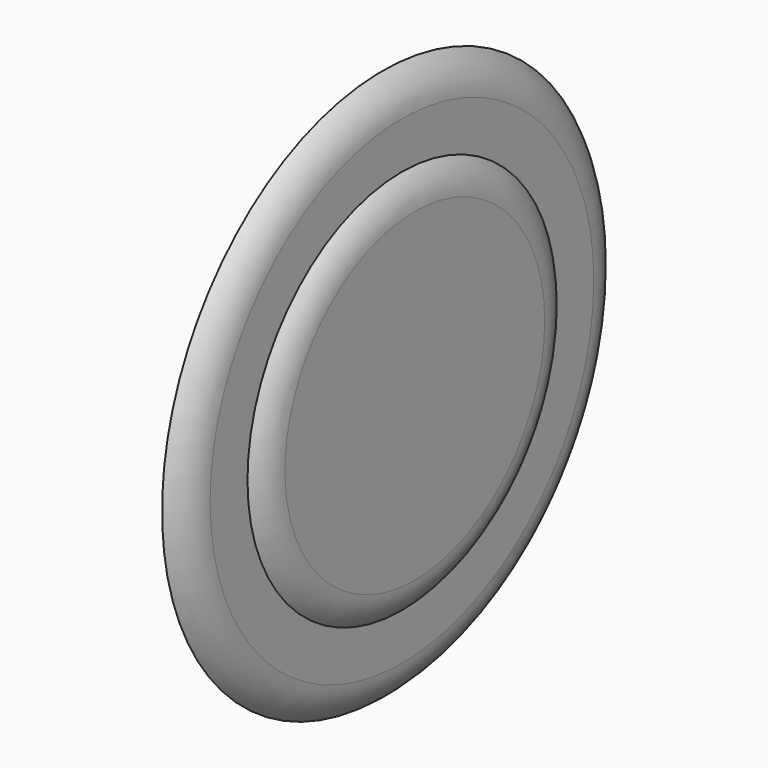
from build123d import *

# Parameters (mm, degrees)
F0_R     = 32.6029937505
F1_DEPTH = 2.286
F2_R     = 22.8313061555
F3_DEPTH = 1.524
F6_R     = 29.7880355639
F7_DEPTH = 1.016


# Not quite as in the source:
# - a fillet or chamfer that OpenCascade refuses, or shapes differently, is made with other operations: its cross-section is extruded or revolved along the edge and cut away or added


with BuildPart() as f1:
    # F0 (on Right) → F1 (new body)
    with BuildSketch(Plane.YZ):
        with Locations((-40.8581867814, 32.8951068223)):
            Circle(F0_R)
    extrude(amount=F1_DEPTH)

    # F2 (on face) → F3 (join)
    with BuildSketch(Plane.YZ.offset(2.286)):
        with Locations((-40.8581867814, 32.8951068223)):
            Circle(F2_R)
    extrude(amount=F3_DEPTH)

    # F4: fillet of radius 5.08 on 1 edges, made by hand

    # F4_s1 → F4_t2 (revolve, cut)
    with BuildSketch(Plane.XY.offset(32.8951068223)):
        with BuildLine():
            ThreePointArc((2.286, -18.0268806259), (3.4135285843, -19.6872507278), (3.81, -21.6547262676))
            Line((3.81, -21.6547262676), (3.81, -18.0268806259))
            Line((3.81, -18.0268806259), (2.286, -18.0268806259))
        make_face()
    revolve(axis=Axis((3.81, -40.8581867814, 32.8951068223), (1, 0, 0)), mode=Mode.SUBTRACT)

    # F5: fillet of radius 5.08 on 1 edges, made by hand

    # F5_s1 → F5_t2 (revolve, cut)
    with BuildSketch(Plane.XY.offset(32.8951068223)):
        with BuildLine():
            ThreePointArc((0, -8.2551930309), (1.6781314829, -10.0881738983), (2.286, -12.4978294754))
            Line((2.286, -12.4978294754), (2.286, -8.2551930309))
            Line((2.286, -8.2551930309), (0, -8.2551930309))
        make_face()
    revolve(axis=Axis((2.286, -40.8581867814, 32.8951068223), (1, 0, 0)), mode=Mode.SUBTRACT)

    # F6 (on face) → F7 (cut)
    with BuildSketch(Plane(origin=(0, 0, 0), x_dir=(0, -1, 0), z_dir=(-1, 0, 0))):
        with Locations((40.8581867814, 32.8951068223)):
            Circle(F6_R)
    extrude(amount=-F7_DEPTH, mode=Mode.SUBTRACT)

    # F8: fillet of radius 5.08 on 1 edges, made by hand

    # F8_s1 → F8_t2 (revolve)
    with BuildSketch(Plane.XY.offset(32.8951068223)):
        with BuildLine():
            ThreePointArc((0, -70.6462223453), (0.7553111541, -69.2046593967), (1.016, -67.5982223453))
            Line((1.016, -67.5982223453), (1.016, -70.6462223453))
            Line((1.016, -70.6462223453), (0, -70.6462223453))
        make_face()
    revolve(axis=Axis((1.016, -40.8581867814, 32.8951068223), (-1, 0, 0)))


solid = f1.part
